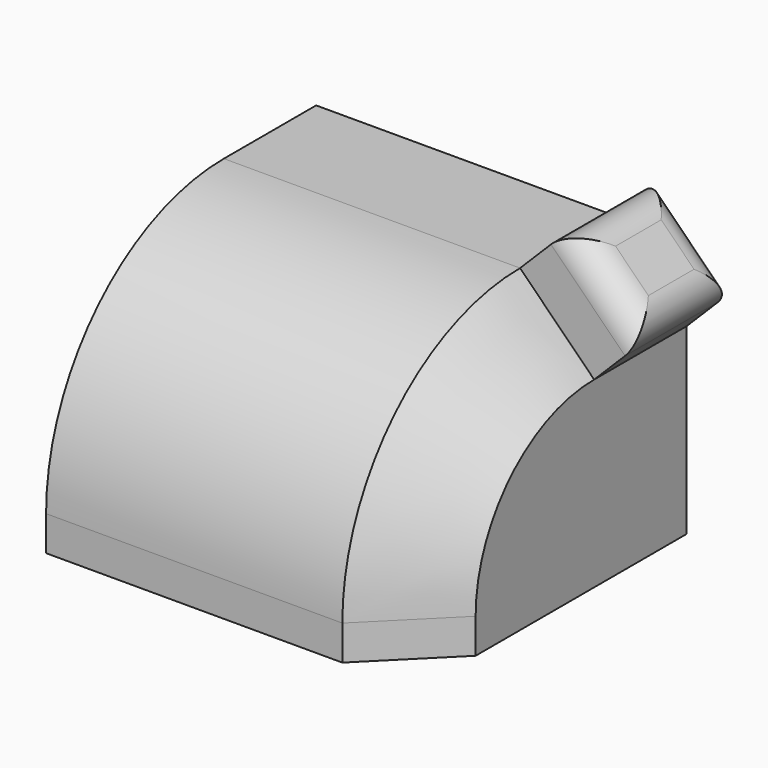
from build123d import *

# Parameters (mm, degrees)
F0_W     = 127
F0_H     = 115.7713381711
F1_DEPTH = 88.138
F2_R     = 76.2
F3_SIZE  = 25.4
F4_DEPTH = 25
F5_R     = 10


# Not quite as in the source:
# - a feature of the source that left no trace in its solid (it failed there, or was rolled back) is left out


with BuildPart() as f1:
    # F0 (on Top) → F1 (new body)
    with BuildSketch(Plane.XY):
        with Locations((0.6131026894, 1.0218378156)):
            Rectangle(F0_W, F0_H)
    extrude(amount=F1_DEPTH)

    # F2
    f2_edges = [f1.edges().sort_by_distance(p)[0] for p in [
        (0.613103, -56.863831, 88.138),
    ]]
    fillet(f2_edges, radius=F2_R)

    # F3
    f3_edges = [f1.edges().sort_by_distance(p)[0] for p in [
        (64.113103, 39.121838, 88.138),
        (64.113103, -56.863831, 5.969),
        (64.113103, -34.545368, 65.819537),
    ]]
    chamfer(f3_edges, length=F3_SIZE)

    # F4 (add): a face of the model
    f4_faces = [f1.faces().sort_by_distance(p)[0] for p in [
        (51.4131026894, 39.1218378156, 75.438),
    ]]
    extrude(f4_faces, amount=F4_DEPTH)

    # F5
    f5_edges = [f1.edges().sort_by_distance(p)[0] for p in [
        (69.090772, 58.907507, 93.11567),
        (69.090772, 19.336169, 93.11567),
        (56.390772, 39.121838, 105.81567),
        (81.790772, 39.121838, 80.41567),
    ]]
    fillet(f5_edges, radius=F5_R)


solid = f1.part
